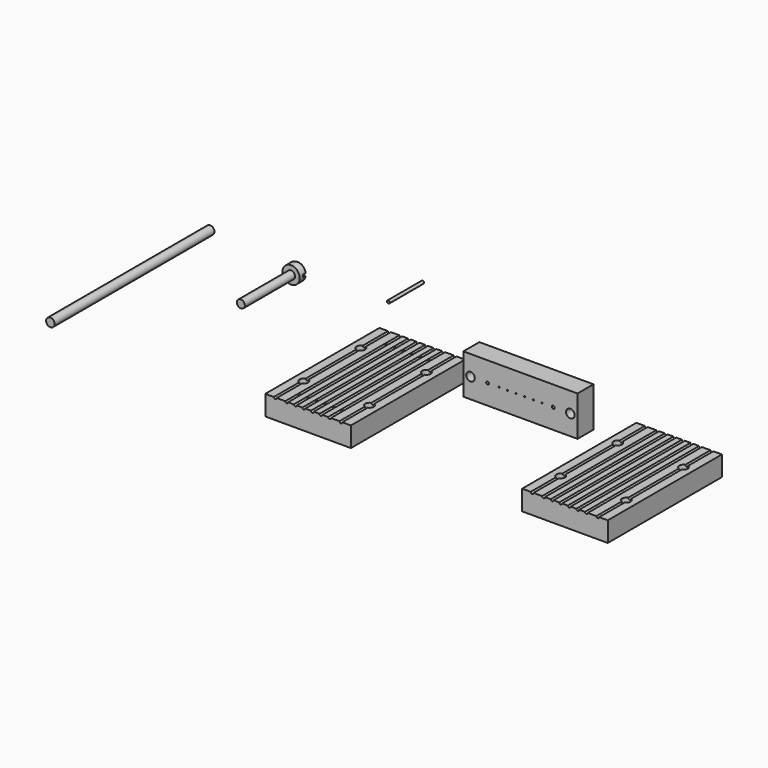
from build123d import *

# Parameters (mm, degrees)
F1_DEPTH  = 50
F2_R      = 0.5
F2_R_2    = 0.2
F2_R_3    = 1.5
F3_DEPTH  = 7
F4_R      = 3
F4_R_2    = 1.4
F5_DEPTH  = 3
F6_DEPTH  = 25
F8_DEPTH  = 1.5
F9_R      = 0.5
F10_R     = 1.5
F10_R_2   = 0.5
F12_DEPTH = 25
F13_R     = 1.5
F14_DEPTH = 25
F15_R     = 0.5
F16_DEPTH = 15
F17_R     = 1.5
F18_DEPTH = 70


# Not quite as in the source:
# - a feature names something its author has since deleted; it is built from what else it names


with BuildPart() as f1:
    # F0 (on Front) → F1 (new body)
    with BuildSketch(Plane.XZ):
        with BuildLine():
            Line((0, 7), (0, 0))
            Line((0, 0), (30, 0))
            Line((30, 0), (30, 7))
            Line((30, 7), (27, 7))
            ThreePointArc((27, 7), (26.5, 6.5), (26, 7))
            Line((26, 7), (23, 7))
            ThreePointArc((23, 7), (22.5, 6.5), (22, 7))
            Line((22, 7), (20, 7))
            ThreePointArc((20, 7), (19.5, 6.5), (19, 7))
            Line((19, 7), (17, 7))
            ThreePointArc((17, 7), (16.5, 6.5), (16, 7))
            Line((16, 7), (14, 7))
            ThreePointArc((14, 7), (13.5, 6.5), (13, 7))
            Line((13, 7), (11, 7))
            ThreePointArc((11, 7), (10.5, 6.5), (10, 7))
            Line((10, 7), (8, 7))
            ThreePointArc((8, 7), (7.5, 6.5), (7, 7))
            Line((7, 7), (4, 7))
            ThreePointArc((4, 7), (3.5, 6.5), (3, 7))
            Line((3, 7), (0, 7))
        make_face()
    extrude(amount=F1_DEPTH)


with BuildPart() as f3:
    # F2 (on Front) → F3 (new body)
    with BuildSketch(Plane.XZ):
        Polygon((40, 7), (40, 0), (70, 0), (70, 7), (70, 14), (40, 14), align=None)
        with Locations((43.5, 7)):
            Circle(F2_R, mode=Mode.SUBTRACT)
        with Locations((47.5, 7)):
            Circle(F2_R_2, mode=Mode.SUBTRACT)
        with Locations((50.5, 7)):
            Circle(F2_R_2, mode=Mode.SUBTRACT)
        with Locations((53.5, 7)):
            Circle(F2_R_2, mode=Mode.SUBTRACT)
        with Locations((56.5, 7)):
            Circle(F2_R_2, mode=Mode.SUBTRACT)
        with Locations((59.5, 7)):
            Circle(F2_R_2, mode=Mode.SUBTRACT)
        with Locations((62.5, 7)):
            Circle(F2_R_2, mode=Mode.SUBTRACT)
        with Locations((66.5, 7)):
            Circle(F2_R, mode=Mode.SUBTRACT)
        Polygon((70, 7), (70, 0), (75, 0), (75, 14), (70, 14), align=None)
        with Locations((72.5, 7)):
            Circle(F2_R_3, mode=Mode.SUBTRACT)
        Polygon((35, 0), (40, 0), (40, 7), (40, 14), (35, 14), align=None)
        with Locations((37.5, 7)):
            Circle(F2_R_3, mode=Mode.SUBTRACT)
    extrude(amount=F3_DEPTH)


with BuildPart() as f5:
    # F4 (on Front) → F5 (new body)
    with BuildSketch(Plane.XZ):
        with Locations((-28.5615846515, 15.2765717357)):
            Circle(F4_R)
        with Locations((-28.5615846515, 15.2765717357)):
            Circle(F4_R_2, mode=Mode.SUBTRACT)
        with Locations((-28.5615846515, 15.2765717357)):
            Circle(F4_R_2)
    extrude(amount=F5_DEPTH)

    # F4 (on Front) → F6 (join)
    with BuildSketch(Plane.XZ):
        with Locations((-28.5615846515, 15.2765717357)):
            Circle(F4_R_2)
    extrude(amount=F6_DEPTH)

    # F7 (on face) → F8 (cut)
    with BuildSketch(Plane.XZ):
        with BuildLine():
            ThreePointArc((-29.8908109833, 14.8370750248), (-29.9615846515, 15.2765717357), (-29.8908109833, 15.7160684466))
            Line((-29.8908109833, 15.7160684466), (-31.5292171491, 15.7160684466))
            ThreePointArc((-31.5292171491, 15.7160684466), (-31.5615846515, 15.2765717357), (-31.5292171491, 14.8370750248))
            Line((-31.5292171491, 14.8370750248), (-29.8908109833, 14.8370750248))
        make_face()
        with BuildLine():
            ThreePointArc((-27.2323583197, 14.8370750248), (-27.1793913103, 15.0539923842), (-27.1615846515, 15.2765717357))
            ThreePointArc((-27.1615846515, 15.2765717357), (-27.1793913103, 15.4991510873), (-27.2323583197, 15.7160684466))
            Line((-27.2323583197, 15.7160684466), (-29.8908109833, 15.7160684466))
            ThreePointArc((-29.8908109833, 15.7160684466), (-29.9615846515, 15.2765717357), (-29.8908109833, 14.8370750248))
            Line((-29.8908109833, 14.8370750248), (-27.2323583197, 14.8370750248))
        make_face()
        with BuildLine():
            ThreePointArc((-27.2323583197, 15.7160684466), (-27.1793913103, 15.4991510873), (-27.1615846515, 15.2765717357))
            ThreePointArc((-27.1615846515, 15.2765717357), (-27.1793913103, 15.0539923842), (-27.2323583197, 14.8370750248))
            Line((-27.2323583197, 14.8370750248), (-25.5939521538, 14.8370750248))
            ThreePointArc((-25.5939521538, 14.8370750248), (-25.5696874697, 15.0562282459), (-25.5615846515, 15.2765717357))
            ThreePointArc((-25.5615846515, 15.2765717357), (-25.5696874697, 15.4969152256), (-25.5939521538, 15.7160684466))
            Line((-25.5939521538, 15.7160684466), (-27.2323583197, 15.7160684466))
        make_face()
    extrude(amount=F8_DEPTH, mode=Mode.SUBTRACT)

    # F9
    f9_edges = [f5.edges().sort_by_distance(p)[0] for p in [
        (-28.561585, 0, 15.716068),
        (-28.561585, 0, 18.276572),
        (-28.561585, 0, 12.276572),
        (-28.561585, 0, 14.837075),
    ]]
    fillet(f9_edges, radius=F9_R)


with BuildPart() as f11_1:
    # F11: copy of F1
    add(f1.part.moved(Location((90, 0, 0))))

    # F13 (on face) → F14 (cut)
    with BuildSketch(Plane(origin=(0, 0, 0), x_dir=(1, 0, 0), z_dir=(0, 0, -1))):
        with Locations((116.5, 37.5)):
            Circle(F13_R)
        with Locations((116.5, 12.5)):
            Circle(F13_R)
        with Locations((93.5, 37.5)):
            Circle(F13_R)
        with Locations((93.5, 12.5)):
            Circle(F13_R)
    extrude(amount=-F14_DEPTH, mode=Mode.SUBTRACT)


with BuildPart() as f1_1:
    add(f1.part)

    # F10 (on face) → F12 (cut)
    with BuildSketch(Plane(origin=(0, 0, 0), x_dir=(1, 0, 0), z_dir=(0, 0, -1))):
        with Locations((3.5, 12.5)):
            Circle(F10_R)
        with Locations((3.5, 37.5)):
            Circle(F10_R)
        with Locations((26.5, 12.5)):
            Circle(F10_R)
        with Locations((26.5, 37.5)):
            Circle(F10_R)
        with Locations((7.5, 6)):
            Circle(F10_R_2)
        with Locations((7.5, 44)):
            Circle(F10_R_2)
        with Locations((10.5, 6)):
            Circle(F10_R_2)
        with Locations((10.5, 44)):
            Circle(F10_R_2)
        with Locations((13.5, 6)):
            Circle(F10_R_2)
        with Locations((13.5, 44)):
            Circle(F10_R_2)
        with Locations((16.5, 6)):
            Circle(F10_R_2)
        with Locations((16.5, 44)):
            Circle(F10_R_2)
        with Locations((19.5, 6)):
            Circle(F10_R_2)
        with Locations((19.5, 44)):
            Circle(F10_R_2)
        with Locations((22.5, 6)):
            Circle(F10_R_2)
        with Locations((22.5, 44)):
            Circle(F10_R_2)
    extrude(amount=-F12_DEPTH, mode=Mode.SUBTRACT)


with BuildPart() as f16:
    # F15 (on Front) → F16 (new body)
    with BuildSketch(Plane.XZ):
        with Locations((15.1483891532, 26.0315593332)):
            Circle(F15_R)
    extrude(amount=F16_DEPTH)


with BuildPart() as f18:
    # F17 (on Front) → F18 (new body)
    with BuildSketch(Plane.XZ):
        with Locations((-59.313505888, 17.875559628)):
            Circle(F17_R)
    extrude(amount=F18_DEPTH)


solid = Compound([f3.part, f5.part, f11_1.part, f1_1.part, f16.part, f18.part])
